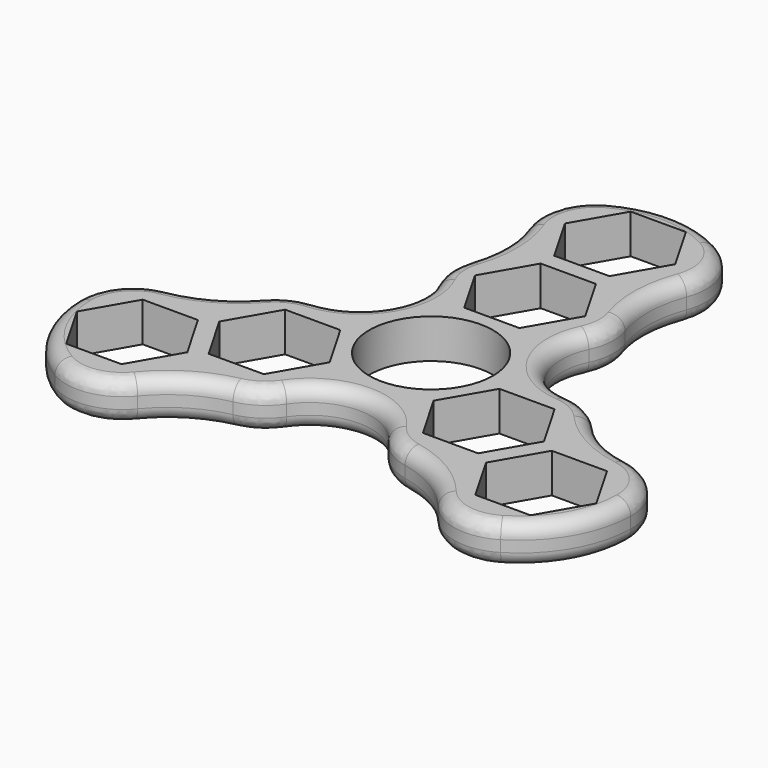
from build123d import *

# Parameters (mm, degrees)
F0_R     = 11
F1_DEPTH = 7
F2_R     = 10
F3_R     = 2.5


# Not quite as in the source:
# - a feature names something its author has since deleted; it is built from what else it names


with BuildPart() as f1:
    # F0 (on Top) → F1 (new body)
    with BuildSketch(Plane.XY):
        with BuildLine():
            ThreePointArc((-15.0856038079, 20.7220792519), (-13.8564064606, 8), (-25.4886489553, 2.7034765031))
            ThreePointArc((-25.4886489553, 2.7034765031), (-26.0562435375, 2.8057189987), (-26.6265501378, 2.8915532538))
            ThreePointArc((-26.6265501378, 2.8915532538), (-35.1569027382, -5.3553303135), (-46.8584181434, -7.3181194723))
            ThreePointArc((-46.8584181434, -7.3181194723), (-46.6381807639, -26.9265662185), (-29.7668864426, -36.9215207572))
            ThreePointArc((-29.7668864426, -36.9215207572), (-22.2163034662, -27.769105733), (-10.8091164947, -24.5050454613))
            ThreePointArc((-10.8091164947, -24.5050454613), (-10.59829784, -23.96822833), (-10.4030451474, -23.425555755))
            ThreePointArc((-10.4030451474, -23.425555755), (0, -16), (10.4030451474, -23.425555755))
            ThreePointArc((10.4030451474, -23.425555755), (10.59829784, -23.96822833), (10.8091164947, -24.5050454613))
            ThreePointArc((10.8091164947, -24.5050454613), (22.2163034662, -27.769105733), (29.7668864426, -36.9215207572))
            ThreePointArc((29.7668864426, -36.9215207572), (46.6381807639, -26.9265662185), (46.8584181434, -7.3181194723))
            ThreePointArc((46.8584181434, -7.3181194723), (35.1569027382, -5.3553303135), (26.6265501378, 2.8915532538))
            ThreePointArc((26.6265501378, 2.8915532538), (26.0562435375, 2.8057189987), (25.4886489553, 2.7034765031))
            ThreePointArc((25.4886489553, 2.7034765031), (13.8564064606, 8), (15.0856038079, 20.7220792519))
            ThreePointArc((15.0856038079, 20.7220792519), (15.4579456975, 21.1625093313), (15.8174336431, 21.6134922076))
            ThreePointArc((15.8174336431, 21.6134922076), (12.940599272, 33.1244360464), (17.0915317007, 44.2396402295))
            ThreePointArc((17.0915317007, 44.2396402295), (0, 53.853132437), (-17.0915317007, 44.2396402295))
            ThreePointArc((-17.0915317007, 44.2396402295), (-12.940599272, 33.1244360464), (-15.8174336431, 21.6134922076))
            ThreePointArc((-15.8174336431, 21.6134922076), (-15.4579456975, 21.1625093313), (-15.0856038079, 20.7220792519))
        make_face()
        Polygon((-26.5581123827, -21), (-31.4655896708, -29.5), (-41.2805442471, -29.5), (-46.1880215352, -21), (-41.2805442471, -12.5), (-31.4655896708, -12.5), align=None, mode=Mode.SUBTRACT)
        Polygon((-14.1450815951, -19.5), (-23.9600361714, -19.5), (-28.8675134595, -11), (-23.9600361714, -2.5), (-14.1450815951, -2.5), (-9.237604307, -11), align=None, mode=Mode.SUBTRACT)
        Polygon((31.4655896708, -29.5), (26.5581123827, -21), (31.4655896708, -12.5), (41.2805442471, -12.5), (46.1880215352, -21), (41.2805442471, -29.5), align=None, mode=Mode.SUBTRACT)
        Polygon((14.1450815951, -2.5), (23.9600361714, -2.5), (28.8675134595, -11), (23.9600361714, -19.5), (14.1450815951, -19.5), (9.237604307, -11), align=None, mode=Mode.SUBTRACT)
        Circle(F0_R, mode=Mode.SUBTRACT)
        Polygon((-9.8149545762, 22), (-4.9074772881, 30.5), (4.9074772881, 30.5), (9.8149545762, 22), (4.9074772881, 13.5), (-4.9074772881, 13.5), align=None, mode=Mode.SUBTRACT)
        Polygon((9.8149545762, 42), (4.9074772881, 33.5), (-4.9074772881, 33.5), (-9.8149545762, 42), (-4.9074772881, 50.5), (4.9074772881, 50.5), align=None, mode=Mode.SUBTRACT)
    extrude(amount=F1_DEPTH)

    # F2
    f2_edges = [f1.edges().sort_by_distance(p)[0] for p in [
        (26.62655, 2.891553, 3.5),
        (15.817434, 21.613492, 3.5),
        (46.858418, -7.318119, 3.5),
        (17.091532, 44.23964, 3.5),
        (-17.091532, 44.23964, 3.5),
        (-15.817434, 21.613492, 3.5),
        (-26.62655, 2.891553, 3.5),
        (-46.858418, -7.318119, 3.5),
        (-29.766886, -36.921521, 3.5),
        (-10.809116, -24.505045, 3.5),
        (10.809116, -24.505045, 3.5),
        (29.766886, -36.921521, 3.5),
    ]]
    fillet(f2_edges, radius=F2_R)

    # F3
    f3_edges = [f1.edges().sort_by_distance(p)[0] for p in [
        (13.856406, 8, 7),
        (13.856406, 8, 0),
        (0, -16, 7),
        (0, -16, 0),
        (-13.856406, 8, 7),
        (-13.856406, 8, 0),
        (-14.415154, 21.927307, 0),
        (-26.197182, 1.520236, 0),
        (-12.913141, 32.408662, 0),
        (-34.523295, -5.021223, 0),
        (-14.231591, 46.048498, 0),
        (-46.994965, -10.69933, 0),
        (0, 53.853132, 0),
        (-46.638181, -26.926566, 0),
        (14.231591, 46.048498, 0),
        (-32.763374, -35.349168, 0),
        (12.913141, 32.408662, 0),
        (-21.610154, -27.387439, 0),
        (14.415154, 21.927307, 0),
        (-11.782028, -23.447543, 0),
        (26.197182, 1.520236, 0),
        (11.782028, -23.447543, 0),
        (34.523295, -5.021223, 0),
        (21.610154, -27.387439, 0),
        (46.994965, -10.69933, 0),
        (32.763374, -35.349168, 0),
        (46.638181, -26.926566, 0),
        (-14.415154, 21.927307, 7),
        (-26.197182, 1.520236, 7),
        (-12.913141, 32.408662, 7),
        (-34.523295, -5.021223, 7),
        (-14.231591, 46.048498, 7),
        (-46.994965, -10.69933, 7),
        (0, 53.853132, 7),
        (-46.638181, -26.926566, 7),
        (14.231591, 46.048498, 7),
        (-32.763374, -35.349168, 7),
        (12.913141, 32.408662, 7),
        (-21.610154, -27.387439, 7),
        (14.415154, 21.927307, 7),
        (-11.782028, -23.447543, 7),
        (26.197182, 1.520236, 7),
        (11.782028, -23.447543, 7),
        (34.523295, -5.021223, 7),
        (21.610154, -27.387439, 7),
        (46.994965, -10.69933, 7),
        (32.763374, -35.349168, 7),
        (46.638181, -26.926566, 7),
    ]]
    fillet(f3_edges, radius=F3_R)


solid = f1.part
